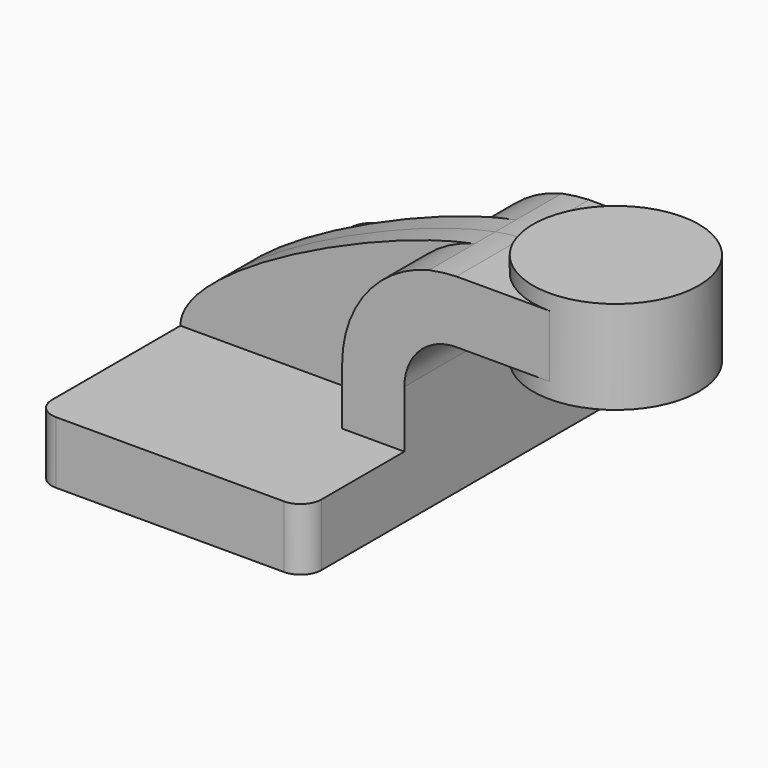
from build123d import *

# Parameters (mm, degrees)
F1_DEPTH = 63.5
F2_DEPTH = 25.4
F3_DEPTH = 7.9375
F0_W     = 25.4
F0_H     = 19.05
F4_DEPTH = 25.4
F6_R     = 6.35


# Not quite as in the source:
# - a feature names something its author has since deleted; it is built from what else it names


with BuildPart() as f1:
    # F0 (on Front) → F1 (new body, symmetric)
    with BuildSketch(Plane.XZ):
        Polygon((-41.275, 9.525), (-41.275, -9.525), (41.275, -9.525), (41.275, 9.525), (22.225, 9.525), align=None)
    extrude(amount=F1_DEPTH, both=True)

    # F0 (on Front) → F2 (join, symmetric)
    with BuildSketch(Plane.XZ):
        with BuildLine():
            Line((22.225, 9.525), (41.275, 9.525))
            Line((41.275, 9.525), (41.275, 27.0002))
            ThreePointArc((41.275, 27.0002), (45.9246798487, 38.2255201513), (57.15, 42.8752))
            Line((57.15, 42.8752), (60.325, 42.8752))
            Line((60.325, 42.8752), (60.325, 61.9252))
            Line((60.325, 61.9252), (57.15, 61.9252))
            add(Edge.make_bspline(
                [(48.8367454286, 60.9213648301), (51.9709953624, 61.5161426584), (54.7763944368, 61.8635493609), (57.15, 61.9252)],
                knots=[100.9548457495, 100.9548457495, 100.9548457495, 100.9548457495, 111.5045361635, 111.5045361635, 111.5045361635, 111.5045361635], degree=3))
            ThreePointArc((48.8367454286, 60.9213648301), (29.6718628642, 48.5572778295), (22.225, 27.0002))
            Line((22.225, 27.0002), (22.225, 9.525))
        make_face()
    extrude(amount=F2_DEPTH, both=True)

    # F0 (on Front) → F3 (join, symmetric)
    with BuildSketch(Plane.XZ):
        with BuildLine():
            add(Edge.make_bspline(
                [(-41.275, 9.525), (-41.2637939453, 26.8850534088), (18.8436644761, 55.2296618934), (48.8367454286, 60.9213648301)],
                knots=[0, 0, 0, 0, 100.9548457495, 100.9548457495, 100.9548457495, 100.9548457495], degree=3))
            Line((-41.275, 9.525), (22.225, 9.525))
            Line((22.225, 9.525), (22.225, 27.0002))
            ThreePointArc((22.225, 27.0002), (29.6718628642, 48.5572778295), (48.8367454286, 60.9213648301))
        make_face()
    extrude(amount=F3_DEPTH, both=True)

    # F0 (on Front) → F4 (join, symmetric)
    with BuildSketch(Plane.XZ):
        with Locations((73.025, 52.4002)):
            Rectangle(F0_W, F0_H)
    extrude(amount=F4_DEPTH, both=True)

    # F0 (on Front) → F5 (revolve)
    with BuildSketch(Plane.XZ):
        Polygon((85.725, 66.675), (85.725, 61.9252), (85.725, 42.8752), (85.725, 38.1), (111.125, 38.1), (111.125, 66.675), align=None)
    revolve(axis=Axis((85.725, 0, 52.3875), (0, 0, 1)))

    # F6
    f6_edges = [f1.edges().sort_by_distance(p)[0] for p in [
        (41.275, 63.5, 0),
        (41.275, -63.5, 0),
        (-41.275, -63.5, 0),
        (-41.275, 63.5, 0),
    ]]
    fillet(f6_edges, radius=F6_R)


solid = f1.part
